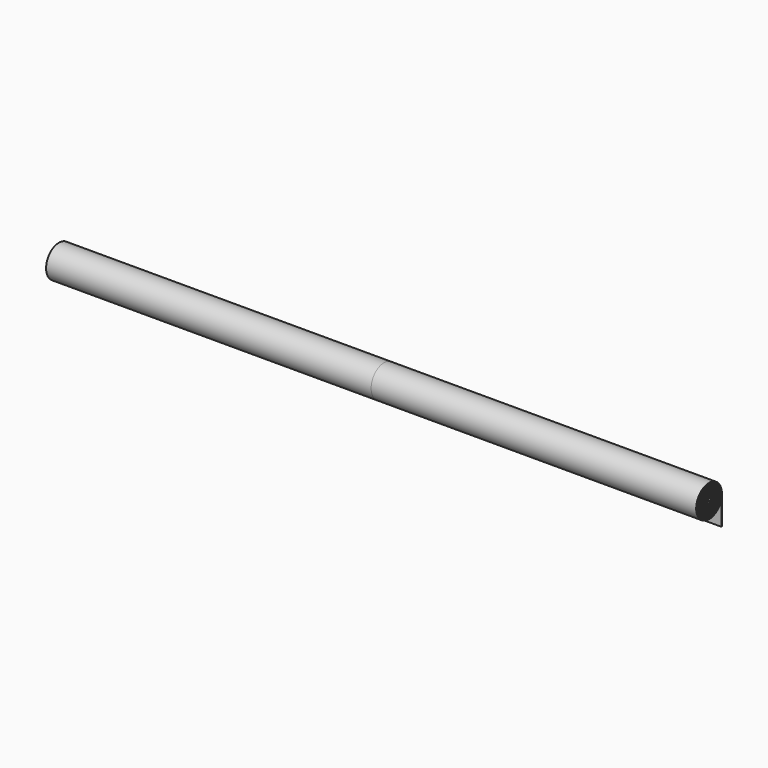
from build123d import *

# Parameters (mm, degrees)
F1_DEPTH      = 641.35
F2_R          = 31.75
F3_DEPTH      = 641.35
F3_DEPTH_BACK = 641.35
F4_R          = 1.27
F5_DEPTH      = 1282.701


# Not quite as in the source:
# - ends of sketch curves that miss each other by under 0.0002 mm in the source are joined


with BuildPart() as f1:
    # F0 (on Right) → F1 (new body, symmetric)
    with BuildSketch(Plane.YZ):
        Polygon((-1.27, 0), (0, 0), (0, 57.15), (-1.27, 57.15), (-1.27, 52.07), align=None)
    extrude(amount=F1_DEPTH, both=True)

    # F2 (on Right) → F3 (join, two sides)
    with BuildSketch(Plane.YZ) as f3_sk:
        with Locations((-31.75, 57.15)):
            Circle(F2_R)
    extrude(amount=F3_DEPTH)
    extrude(f3_sk.sketch, amount=-F3_DEPTH_BACK)

    # F4 (on face) → F5 (cut, through all)
    with BuildSketch(Plane.YZ.offset(641.35)):
        with BuildLine():
            ThreePointArc((-62.2299973542, 57.1373), (-31.7436499999, 26.6700006615), (-1.27, 57.15))
            ThreePointArc((-1.27, 57.15), (-31.7436499999, 87.6299993385), (-62.2299973542, 57.1627))
            Line((-62.2299973542, 57.1627), (-61.5949972979, 57.1627))
            ThreePointArc((-61.5949972979, 57.1627), (-31.7436499999, 86.9949993245), (-1.905, 57.15))
            ThreePointArc((-1.905, 57.15), (-31.7436499999, 27.3050006755), (-61.5949972979, 57.1373))
            Line((-61.5949972979, 57.1373), (-62.2299973542, 57.1373))
        make_face()
        with BuildLine():
            ThreePointArc((-3.175, 57.15), (-31.7436499998, 85.7249992944), (-60.3249971778, 57.1627))
            Line((-60.3249971778, 57.1627), (-59.6899971136, 57.1627))
            ThreePointArc((-59.6899971136, 57.1627), (-31.7436499998, 85.0899992784), (-3.81, 57.15))
            ThreePointArc((-3.81, 57.15), (-31.7436499998, 29.2100007216), (-59.6899971136, 57.1373))
            Line((-59.6899971136, 57.1373), (-60.3249971778, 57.1373))
            ThreePointArc((-60.3249971778, 57.1373), (-31.7436499998, 28.5750007056), (-3.175, 57.15))
        make_face()
        with BuildLine():
            ThreePointArc((-5.08, 57.15), (-31.7436499998, 83.819999244), (-58.4199969762, 57.1627))
            Line((-58.4199969762, 57.1627), (-57.7849969024, 57.1627))
            ThreePointArc((-57.7849969024, 57.1627), (-31.7436499998, 83.1849992256), (-5.715, 57.15))
            ThreePointArc((-5.715, 57.15), (-31.7436499998, 31.1150007744), (-57.7849969024, 57.1373))
            Line((-57.7849969024, 57.1373), (-58.4199969762, 57.1373))
            ThreePointArc((-58.4199969762, 57.1373), (-31.7436499998, 30.480000756), (-5.08, 57.15))
        make_face()
        with BuildLine():
            ThreePointArc((-6.985, 57.15), (-31.7436499998, 81.9149991859), (-56.5149967436, 57.1626999999))
            Line((-56.5149967436, 57.1626999999), (-55.8799969024, 57.1627))
            ThreePointArc((-55.8799969024, 57.1627), (-31.7436499998, 81.279999409), (-7.6199997555, 57.15))
            ThreePointArc((-7.6199997555, 57.15), (-31.7436499998, 33.020000591), (-55.8799969024, 57.1373))
            Line((-55.8799969024, 57.1373), (-56.5149969762, 57.1373))
            ThreePointArc((-56.5149969762, 57.1373), (-31.7436499998, 32.3850008141), (-6.985, 57.15))
        make_face()
        with BuildLine():
            ThreePointArc((-8.8899997286, 57.15), (-31.7436499998, 80.0099993894), (-54.6099967436, 57.1626999999))
            Line((-54.6099967436, 57.1626999999), (-53.9749969024, 57.1627))
            ThreePointArc((-53.9749969024, 57.1627), (-31.7436499997, 79.3749996239), (-9.524999469, 57.15))
            ThreePointArc((-9.524999469, 57.15), (-31.7436499997, 34.9250003761), (-53.9749969024, 57.1373))
            Line((-53.9749969024, 57.1373), (-54.6099969762, 57.1373))
            ThreePointArc((-54.6099969762, 57.1373), (-31.7436499998, 34.2900006106), (-8.8899997286, 57.15))
        make_face()
        with BuildLine():
            ThreePointArc((-10.7949994079, 57.15), (-31.7436499997, 78.10499963), (-52.7049967436, 57.1626999999))
            Line((-52.7049967436, 57.1626999999), (-52.0699969024, 57.1627))
            ThreePointArc((-52.0699969024, 57.1627), (-31.7436499997, 77.469999879), (-11.4299991288, 57.15))
            ThreePointArc((-11.4299991288, 57.15), (-31.7436499997, 36.830000121), (-52.0699969024, 57.1373))
            Line((-52.0699969024, 57.1373), (-52.7049969762, 57.1373))
            ThreePointArc((-52.7049969762, 57.1373), (-31.7436499997, 36.19500037), (-10.7949994079, 57.15))
        make_face()
        with BuildLine():
            ThreePointArc((-12.6999987905, 57.15), (-31.7436499996, 76.2000001512), (-50.7999969762, 57.1627000001))
            Line((-50.7999969762, 57.1627), (-50.1649969024, 57.1627))
            ThreePointArc((-50.1649969024, 57.1627), (-31.7436499996, 75.5650001869), (-13.3349987183, 57.15))
            ThreePointArc((-13.3349987183, 57.15), (-31.7436499996, 38.7349998131), (-50.1649969024, 57.1373))
            Line((-50.1649969024, 57.1373), (-50.7999969762, 57.1373))
            ThreePointArc((-50.7999969762, 57.1372999999), (-31.7436499996, 38.0999998488), (-12.6999987905, 57.15))
        make_face()
        with BuildLine():
            ThreePointArc((-14.6049985527, 57.15), (-31.7436499996, 74.2950002714), (-48.8949967436, 57.1626999999))
            Line((-48.8949967436, 57.1626999999), (-48.2599969024, 57.1627))
            ThreePointArc((-48.2599969024, 57.1627), (-31.7436499995, 73.6600005659), (-15.2399982129, 57.15))
            ThreePointArc((-15.2399982129, 57.15), (-31.7436499995, 40.6399994341), (-48.2599969024, 57.1373))
            Line((-48.2599969024, 57.1373), (-48.8949969762, 57.1373))
            ThreePointArc((-48.8949969762, 57.1373), (-31.7436499996, 40.0049997286), (-14.6049985527, 57.15))
        make_face()
        with BuildLine():
            ThreePointArc((-16.5099979647, 57.15), (-31.7436499995, 72.3900007123), (-46.9899967436, 57.1626999999))
            Line((-46.9899967436, 57.1626999999), (-46.3549969024, 57.1627))
            ThreePointArc((-46.3549969024, 57.1627), (-31.7436499994, 71.7550010437), (-17.1449975758, 57.15))
            ThreePointArc((-17.1449975758, 57.15), (-31.7436499994, 42.5449989563), (-46.3549969024, 57.1373))
            Line((-46.3549969024, 57.1373), (-46.9899969762, 57.1373))
            ThreePointArc((-46.9899969762, 57.1373), (-31.7436499995, 41.9099992877), (-16.5099979647, 57.15))
        make_face()
        with BuildLine():
            ThreePointArc((-18.4149972088, 57.15), (-31.7436499993, 70.4850012793), (-45.0849967436, 57.1626999999))
            Line((-45.0849967436, 57.1626999999), (-44.4499969024, 57.1627))
            ThreePointArc((-44.4499969024, 57.1627), (-31.7436499992, 69.8500016649), (-19.0499967476, 57.15))
            ThreePointArc((-19.0499967476, 57.15), (-31.7436499992, 44.4499983351), (-44.4499969024, 57.1373))
            Line((-44.4499969024, 57.1373), (-45.0849969762, 57.1373))
            ThreePointArc((-45.0849969762, 57.1373), (-31.7436499993, 43.8149987207), (-18.4149972088, 57.15))
        make_face()
        with BuildLine():
            ThreePointArc((-20.3199959683, 57.15), (-31.743649999, 68.5800022679), (-43.1799969762, 57.1627000001))
            Line((-43.1799969762, 57.1627), (-42.5449969024, 57.1627))
            ThreePointArc((-42.5449969024, 57.1627), (-31.7436499989, 67.9450025054), (-20.954995627, 57.15))
            ThreePointArc((-20.954995627, 57.15), (-31.7436499989, 46.3549974946), (-42.5449969024, 57.1373))
            Line((-42.5449969024, 57.1373), (-43.1799969762, 57.1373))
            ThreePointArc((-43.1799969762, 57.1372999999), (-31.743649999, 45.7199977321), (-20.3199959683, 57.15))
        make_face()
        with BuildLine():
            ThreePointArc((-22.2249947897, 57.15), (-31.7436499987, 66.6750030936), (-41.2749967436, 57.1626999998))
            Line((-41.2749967436, 57.1626999998), (-40.6399969024, 57.1627))
            ThreePointArc((-40.6399969024, 57.1627), (-31.7436499984, 66.040003706), (-22.8599940261, 57.15))
            ThreePointArc((-22.8599940261, 57.15), (-31.7436499984, 48.259996294), (-40.6399969024, 57.1373))
            Line((-40.6399969024, 57.1373), (-41.2749969762, 57.1373))
            ThreePointArc((-41.2749969762, 57.1373), (-31.7436499987, 47.6249969064), (-22.2249947897, 57.15))
        make_face()
        with BuildLine():
            ThreePointArc((-24.1299926731, 57.15), (-31.7436499979, 64.7700046811), (-39.3699967436, 57.1626999998))
            Line((-39.3699967436, 57.1626999998), (-38.7349969024, 57.1627))
            ThreePointArc((-38.7349969024, 57.1627), (-31.7436499974, 64.1350055615), (-24.7649915521, 57.15))
            ThreePointArc((-24.7649915521, 57.15), (-31.7436499974, 50.1649944385), (-38.7349969024, 57.1373))
            Line((-38.7349969024, 57.1373), (-39.3699969762, 57.1373))
            ThreePointArc((-39.3699969762, 57.1373), (-31.7436499979, 49.5299953189), (-24.1299926731, 57.15))
        make_face()
        with BuildLine():
            ThreePointArc((-26.0349891453, 57.15), (-31.7436499962, 62.8650073269), (-37.4649967436, 57.1626999997))
            Line((-37.4649967436, 57.1626999997), (-36.8299969024, 57.1627))
            ThreePointArc((-36.8299969024, 57.1627), (-31.743649995, 62.2300088087), (-26.6699872226, 57.15))
            ThreePointArc((-26.6699872226, 57.15), (-31.743649995, 52.0699911913), (-36.8299969024, 57.1373))
            Line((-36.8299969024, 57.1373), (-37.4649969762, 57.1373))
            ThreePointArc((-37.4649969762, 57.1373), (-31.7436499962, 51.4349926731), (-26.0349891453, 57.15))
        make_face()
        with Locations((-31.75, 57.15)):
            Circle(F4_R)
    extrude(amount=-F5_DEPTH, mode=Mode.SUBTRACT)


solid = f1.part
